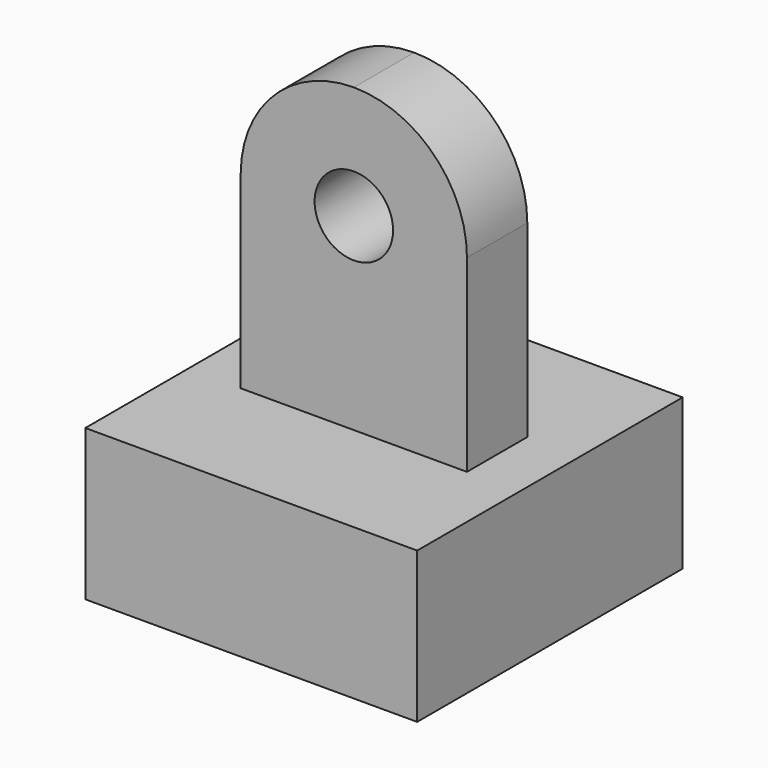
from build123d import *

# Parameters (mm, degrees)
F0_W     = 27.94
F0_H     = 12.7
F1_DEPTH = 27.94
F2_W     = 19.05
F2_H     = 6.35
F3_DEPTH = 25.4
F4_R     = 9.52499
F5_R     = 3.302
F6_DEPTH = 6.35
F7_W     = 1.5875
F7_H     = 12.7
F8_DEPTH = 22.225


# Not quite as in the source:
# - a fillet or chamfer is up to 0.001 mm smaller than in the source, because OpenCascade refuses the exact size


with BuildPart() as f1:
    # F0 (on Front) → F1 (new body)
    with BuildSketch(Plane.XZ):
        with Locations((-13.97, -199.4363271219)):
            Rectangle(F0_W, F0_H)
    extrude(amount=-F1_DEPTH)

    # F2 (on face) → F3 (join)
    with BuildSketch(Plane.XY.offset(-193.0863271219)):
        with Locations((-13.97, 13.97)):
            Rectangle(F2_W, F2_H)
    extrude(amount=F3_DEPTH)

    # F4 (radius 9.525 in the source; OpenCascade refuses exactly that, so slightly less here)
    f4_edges = [f1.edges().sort_by_distance(p)[0] for p in [
        (-4.445, 13.97, -167.686327),
        (-23.495, 13.97, -167.686327),
    ]]
    fillet(f4_edges, radius=F4_R)

    # F5 (on face) → F6 (cut)
    with BuildSketch(Plane.XZ.offset(-10.795)):
        with Locations((-13.97, -177.2113271219)):
            Circle(F5_R)
    extrude(amount=-F6_DEPTH, mode=Mode.SUBTRACT)

    # F7 (on face) → F8 (cut)
    with BuildSketch(Plane(origin=(-27.94, 0, 0), x_dir=(0, -1, 0), z_dir=(-1, 0, 0))):
        with Locations((-25.55875, -177.2113271219)):
            Rectangle(F7_W, F7_H)
    extrude(amount=-F8_DEPTH, mode=Mode.SUBTRACT)


solid = f1.part
